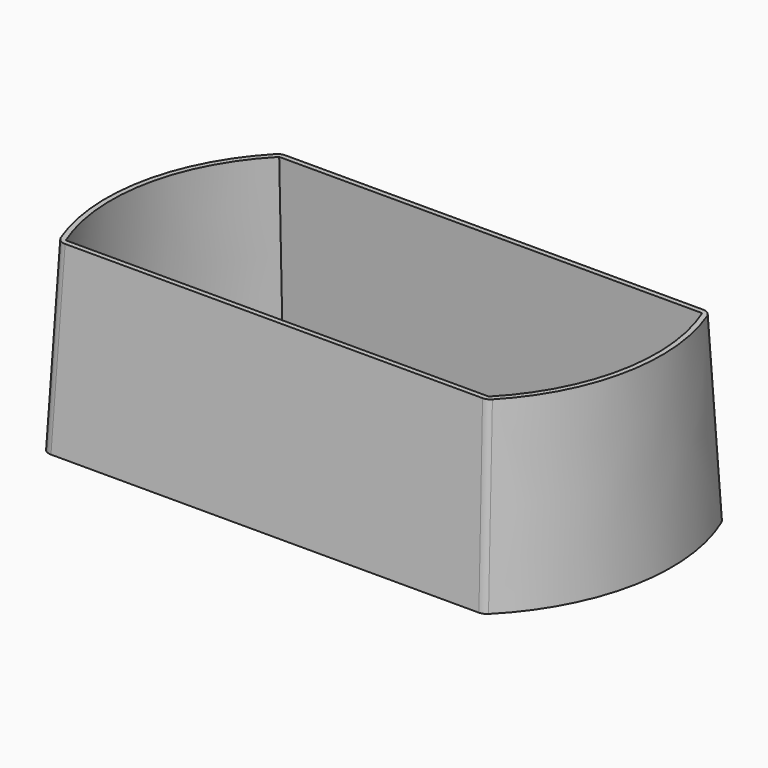
from build123d import *

# Parameters (mm, degrees)
F1_DEPTH               = 90
DRAFT_F1_DRAFTED_ANGLE = -3
F2_T                   = -2.5
F3_R                   = 5


# Not quite as in the source:
# - an extrude with a draft is written as a straight extrude whose walls are then drafted


with BuildPart() as f1:
    # F0 (on Top) → F1 (new body)
    with BuildSketch(Plane.XY):
        with BuildLine():
            Line((139.2598989654, 70.6812429547), (-70.7401010346, 70.6812429547))
            ThreePointArc((-70.7401010346, 70.6812429547), (-98.1920460222, 18.9293977181), (-91.9458283143, -39.3187570453))
            Line((-91.9458283143, -39.3187570453), (118.0541716857, -39.3187570453))
            ThreePointArc((118.0541716857, -39.3187570453), (145.5061166733, 12.4330881913), (139.2598989654, 70.6812429547))
        make_face()
    extrude(amount=-F1_DEPTH)

    # draft_F1_drafted
    draft_f1_drafted_walls = [f1.faces().sort_by_distance(p)[0] for p in [
        (13.0541716857, -39.3187570453, -60),
        (145.5061166733, 12.4330881913, -60),
        (34.2598989654, 70.6812429547, -60),
        (-98.1920460222, 18.9293977181, -60),
    ]]
    draft(draft_f1_drafted_walls, neutral_plane=Plane(origin=(0, 0, 0), x_dir=(1, 0, 0), z_dir=(0, 0, -1)), angle=DRAFT_F1_DRAFTED_ANGLE)

    # F2
    f2_openings = [f1.faces().sort_by_distance(p)[0] for p in [
        (23.657035, 15.681243, 0),
    ]]
    offset(amount=F2_T, openings=f2_openings, kind=Kind.INTERSECTION)

    # F3
    f3_edges = [f1.edges().sort_by_distance(p)[0] for p in [
        (-93.476771, -41.657795, -44.6315),
        (119.018463, -41.661249, -44.697417),
        (140.790842, 73.020281, -44.6315),
        (-71.704392, 73.023735, -44.697417),
    ]]
    fillet(f3_edges, radius=F3_R)


solid = f1.part
